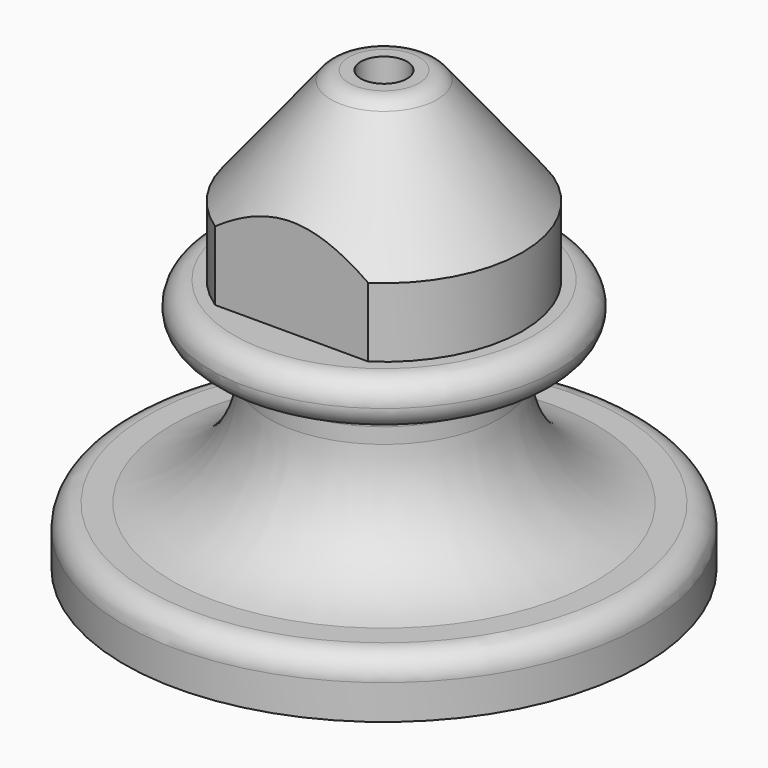
from build123d import *

# Parameters (mm, degrees)
F2_R     = 1.99999
F4_DEPTH = 16.001


# Not quite as in the source:
# - a fillet or chamfer is up to 0.001 mm smaller than in the source, because OpenCascade refuses the exact size


with BuildPart() as f1:
    # F0 (on Front) → F1 (revolve)
    with BuildSketch(Plane.XZ):
        with BuildLine():
            Line((4, 16), (2, 16))
            Line((2, 16), (2, 3))
            Line((2, 3), (7, 3))
            Line((7, 3), (7, -7.3400610127))
            ThreePointArc((7, -7.3400610127), (10.6445666102, -16.2782654993), (19.5, -20.1195757836))
            Line((19.5, -20.1195757836), (19.5, -22))
            Line((19.5, -22), (22.5, -22))
            Line((22.5, -22), (22.5, -17))
            Line((22.5, -17), (18.3448173129, -17))
            ThreePointArc((18.3448173129, -17), (12.4305503735, -13.6747490325), (10, -7.3400610127))
            Line((10, -7.3400610127), (10, -4))
            Line((10, -4), (15, -4))
            Line((15, -4), (15, 0))
            Line((15, 0), (12, 0))
            Line((12, 0), (12, 6))
            Line((12, 6), (4, 16))
        make_face()
    revolve(axis=Axis((0, 0, 9.5), (0, 0, -1)))

    # F2 (radius 2 in the source; OpenCascade refuses exactly that, so slightly less here)
    f2_edges = [f1.edges().sort_by_distance(p)[0] for p in [
        (-4, 0, 16),
        (-15, 0, 0),
        (-15, 0, -4),
        (-22.5, 0, -17),
        (-19.5, 0, -20.119576),
        (-10, 0, -4),
        (-7, 0, 3),
    ]]
    fillet(f2_edges, radius=F2_R)

    # F3 (on Top) → F4 (cut, through all)
    with BuildSketch(Plane.XY):
        with BuildLine():
            Line((-6.6332495807, 10), (6.6332495807, 10))
            ThreePointArc((6.6332495807, 10), (0, 12), (-6.6332495807, 10))
        make_face()
        with BuildLine():
            ThreePointArc((-6.6332495807, -10), (0, -12), (6.6332495807, -10))
            Line((6.6332495807, -10), (-6.6332495807, -10))
        make_face()
    extrude(amount=F4_DEPTH, mode=Mode.SUBTRACT)


solid = f1.part
